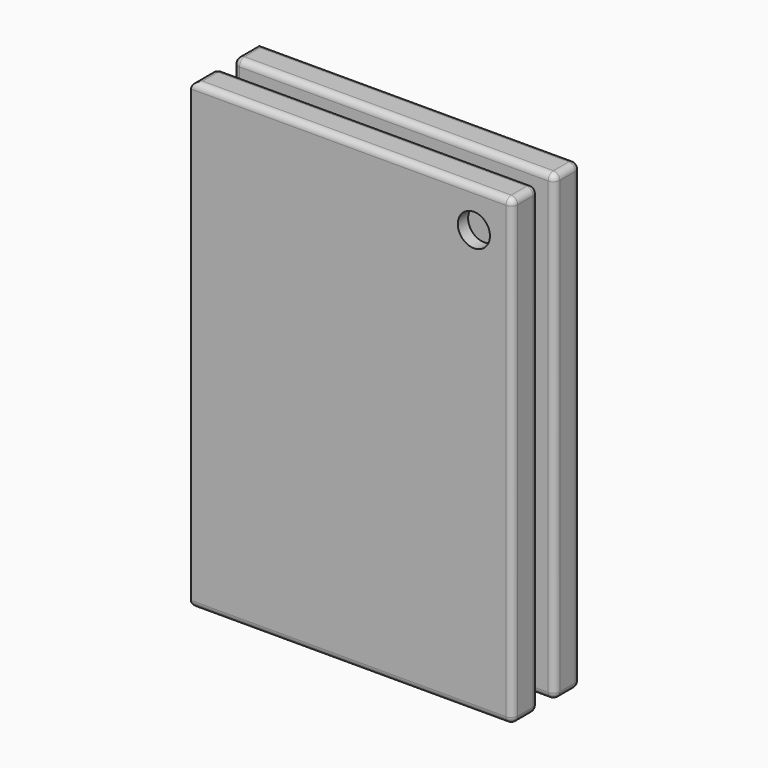
from build123d import *

# Parameters (mm, degrees)
F3_R     = 12.5
F4_DEPTH = 10
F6_DEPTH = 30
F7_R     = 5


with BuildPart() as f2:
    # F2: sweep along a path in F1
    with BuildLine(Plane.XZ) as f2_path:
        Line((0, 0), (250, 0))
    # F0 (on Right) → F2 (sweep)
    with BuildSketch(Plane.YZ):
        Polygon((8, 150), (0, 150), (-8, 150), (-8, 180), (-33, 180), (-33, -180), (-8, -180), (-8, -150), (0, -150), (8, -150), (8, -180), (33, -180), (33, 180), (8, 180), align=None)
    sweep(path=f2_path.line)

    # F3 (on face) → F4 (cut)
    with BuildSketch(Plane.XZ.offset(33)):
        with Locations((220, 150)):
            Circle(F3_R)
    extrude(amount=-F4_DEPTH, mode=Mode.SUBTRACT)

    # F5 (on face) → F6 (cut)
    with BuildSketch(Plane.YZ.offset(250)):
        Polygon((8, 150), (0, 150), (-8, 150), (-8, -150), (0, -150), (8, -150), align=None)
    extrude(amount=-F6_DEPTH, mode=Mode.SUBTRACT)

    # F7
    f7_edges = [f2.edges().sort_by_distance(p)[0] for p in [
        (110, 8, 150),
        (220, 0, 150),
        (110, -8, 150),
        (0, 0, 150),
        (110, -8, -150),
        (220, 0, -150),
        (110, 8, -150),
        (0, 0, -150),
        (125, 33, 180),
        (0, 20.5, 180),
        (125, 8, 180),
        (250, 20.5, 180),
        (125, -8, 180),
        (0, -20.5, 180),
        (125, -33, 180),
        (250, -20.5, 180),
        (125, 8, -180),
        (0, 20.5, -180),
        (125, 33, -180),
        (250, 20.5, -180),
        (125, -33, -180),
        (0, -20.5, -180),
        (125, -8, -180),
        (250, -20.5, -180),
        (0, -8, 165),
        (0, -8, -165),
        (0, 8, -165),
        (0, 8, 165),
        (250, 8, 0),
        (250, 33, 0),
        (250, -8, 0),
        (250, -33, 0),
        (220, -8, 0),
        (220, 8, 0),
    ]]
    fillet(f7_edges, radius=F7_R)


solid = f2.part
